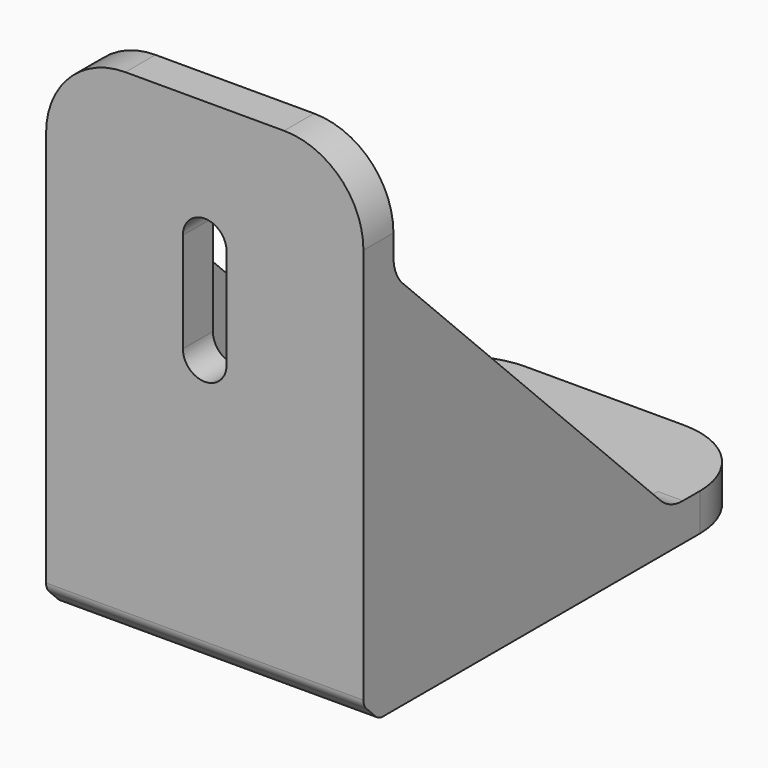
from build123d import *

# Parameters (mm, degrees)
F1_DEPTH        = 12.7
F2_R            = 9.525
F3_SIZE         = 1.524
F4_R            = 1.016
F6_DEPTH        = 2
F7_R            = 6.35
F8_R            = 3.175
F10_DEPTH       = 3.001
F12_D           = 4.4958
F12_DEPTH       = 25.4
F12_CSINK_D     = 9.1186
F12_CSINK_ANGLE = 82
F12_TIP         = 1.3506745855


# Not quite as in the source:
# - a pattern or mirror of a feature is missing from the dataset's text; its kind, count and spacing are read off the source's solid


with BuildPart() as f1:
    # F0 (on Right) → F1 (new body, symmetric)
    with BuildSketch(Plane.YZ):
        Polygon((3, 40), (0, 40), (0, 0), (40, 0), (40, 3), (3, 3), align=None)
    extrude(amount=F1_DEPTH, both=True)

    # F2
    f2_edges = [f1.edges().sort_by_distance(p)[0] for p in [
        (0, 3, 3),
    ]]
    fillet(f2_edges, radius=F2_R)

    # F3
    f3_edges = [f1.edges().sort_by_distance(p)[0] for p in [
        (0, 0, 0),
    ]]
    chamfer(f3_edges, length=F3_SIZE)

    # F4
    f4_edges = [f1.edges().sort_by_distance(p)[0] for p in [
        (0, 0, 1.524),
        (0, 1.524, 0),
    ]]
    fillet(f4_edges, radius=F4_R)

    # F5 (on face) → F6 (join)
    with BuildSketch(Plane.YZ.offset(12.7)):
        with BuildLine():
            Line((33.65, 0), (0, 33.65))
            Line((0, 33.65), (0, 1.9448409794))
            ThreePointArc((0, 1.9448409794), (0.077338395, 1.5560346121), (0.2975795103, 1.2264204897))
            Line((0.2975795103, 1.2264204897), (1.2264204897, 0.2975795103))
            ThreePointArc((1.2264204897, 0.2975795103), (1.5560346121, 0.077338395), (1.9448409794, 0))
            Line((1.9448409794, 0), (33.65, 0))
        make_face()
    f6 = extrude(amount=-F6_DEPTH)

    # F6_copies: F6 across plane
    add(f6.mirror(Plane(origin=(0, 0, 0), x_dir=(0, 0, -1), z_dir=(-1, 0, 0))))

    # F7
    f7_edges = [f1.edges().sort_by_distance(p)[0] for p in [
        (12.7, 1.5, 40),
        (-12.7, 1.5, 40),
        (-12.7, 40, 1.5),
        (12.7, 40, 1.5),
    ]]
    fillet(f7_edges, radius=F7_R)

    # F8
    f8_edges = [f1.edges().sort_by_distance(p)[0] for p in [
        (11.7, 3, 30.65),
        (11.7, 30.65, 3),
        (-11.7, 30.65, 3),
        (-11.7, 3, 30.65),
    ]]
    fillet(f8_edges, radius=F8_R)

    # F9 (on face) → F10 (cut, through all)
    with BuildSketch(Plane(origin=(0, 3, 0), x_dir=(-1, 0, 0), z_dir=(0, 1, 0))):
        with BuildLine():
            Line((1.75, 22), (1.75, 30))
            ThreePointArc((1.75, 30), (0, 28.25), (-1.75, 30))
            Line((-1.75, 30), (-1.75, 22))
            ThreePointArc((-1.75, 22), (0, 23.75), (1.75, 22))
        make_face()
        with BuildLine():
            ThreePointArc((-1.75, 30), (0, 28.25), (1.75, 30))
            ThreePointArc((1.75, 30), (0, 31.75), (-1.75, 30))
        make_face()
        with BuildLine():
            ThreePointArc((-1.75, 22), (0, 20.25), (1.75, 22))
            ThreePointArc((1.75, 22), (0, 23.75), (-1.75, 22))
        make_face()
    extrude(amount=-F10_DEPTH, mode=Mode.SUBTRACT)

    # F12
    with Locations(Plane.XY.offset(3)):
        with Locations((0, 26.2625)):
            CounterSinkHole(F12_D / 2, F12_CSINK_D / 2, depth=F12_DEPTH, counter_sink_angle=F12_CSINK_ANGLE)
            with Locations((0, 0, -(F12_DEPTH + F12_TIP / 2))):  # 118° drill point
                Cone(0, F12_D / 2, F12_TIP, mode=Mode.SUBTRACT)


solid = f1.part
